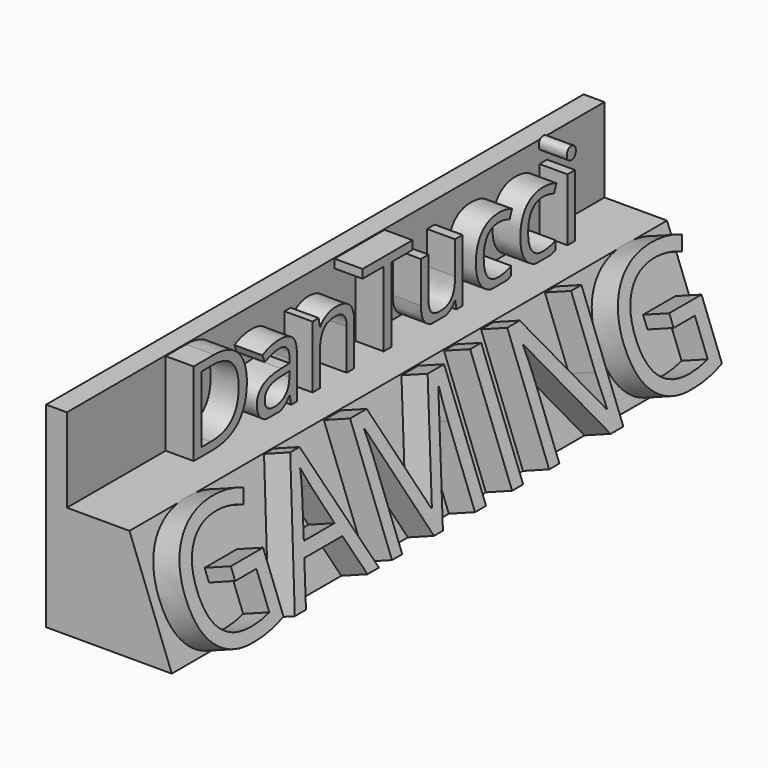
from build123d import *

# Parameters (mm, degrees)
F1_DEPTH     = 609.6
F2_W         = 18.9187638981
F2_H         = 609.6
F3_DEPTH     = 76.2
F5_DEPTH     = 508
F6_TEXT_SIZE = 105.8333333333
F7_DEPTH     = 25.4
F8_TEXT_SIZE = 150.8351191422
F9_DEPTH     = 25.4


# Not quite as in the source:
# - Text() gives the source's letters only with a copy of the font that has no kerning and outlines rounded to 1/6400 em; it was checked with that copy


with BuildPart() as f1:
    # F0 (on Front) → F1 (new body)
    with BuildSketch(Plane.XZ):
        Polygon((37.8375277962, -100.2097258925), (0, -100.2097258925), (0, -201.8097258925), (76.2, -201.8097258925), align=None)
        Polygon((0, -201.8097258925), (0, -100.2097258925), (-37.8375277962, -100.2097258925), (-76.2, -201.8097258925), align=None)
    extrude(amount=F1_DEPTH)

    # F2 (on face) → F3 (join)
    with BuildSketch(Plane.XY.offset(-100.2097258925)):
        with Locations((-28.3781458472, -304.8)):
            Rectangle(F2_W, F2_H)
    extrude(amount=F3_DEPTH)

    # F4 (on face) → F5 (cut)
    with BuildSketch(Plane.XZ.offset(609.6)):
        Polygon((-37.8375277962, -201.8097258925), (-37.8375277962, -100.2097258925), (-76.2, -201.8097258925), align=None)
    extrude(amount=-F5_DEPTH, mode=Mode.SUBTRACT)

    # F6 (on face) → F7 (join)
    with BuildSketch(Plane.YZ.offset(-18.9187638981)):
        with Locations((-508, -100.2097258925)):
            Text('DanTucci', F6_TEXT_SIZE, font='Open Sans', text_align=(TextAlign.LEFT, TextAlign.BOTTOM))
    extrude(amount=F7_DEPTH)

    # F8 (on face) → F9 (join)
    with BuildSketch(Plane(origin=(0, 0, 0), x_dir=(0, 1, 0), z_dir=(0.9355322017, 0, 0.3532414182))):
        with Locations((-609.6, -215.7164932609)):
            Text('GAMING', F8_TEXT_SIZE, font='Open Sans', text_align=(TextAlign.LEFT, TextAlign.BOTTOM))
    extrude(amount=F9_DEPTH)


solid = f1.part
